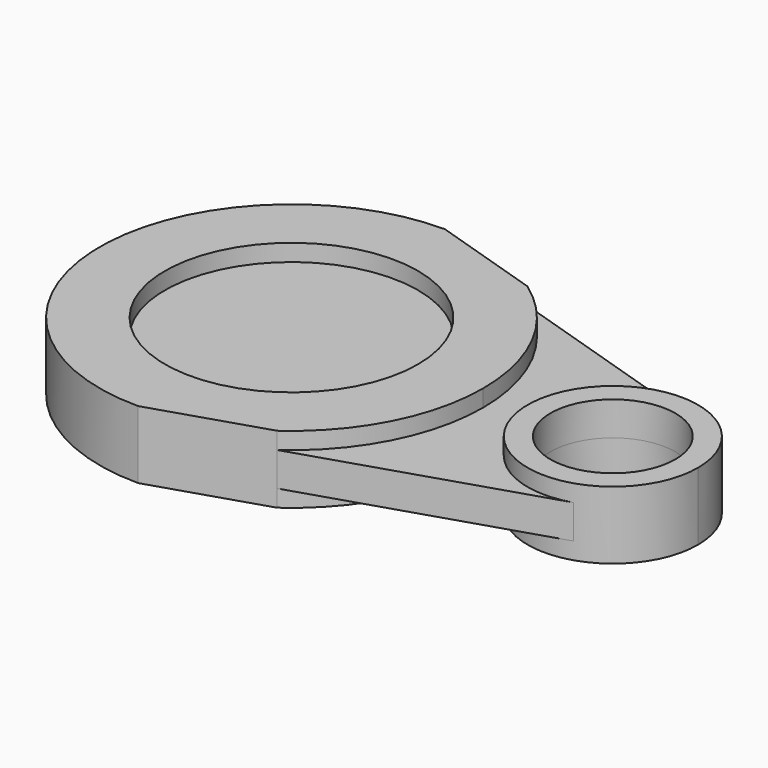
from build123d import *

# Parameters (mm, degrees)
F0_R     = 47.411095877
F1_DEPTH = 12.7
F0_R_2   = 23.4128804589
F2_DEPTH = 6.35


with BuildPart() as f1:
    # F0 (on Top) → F1 (new body, symmetric)
    with BuildSketch(Plane.XY):
        with BuildLine():
            Line((41.5098547303, 58.6180414786), (0, 71.8271733157))
            ThreePointArc((0, 71.8271733157), (-71.8271733157, 0), (0, -71.8271733157))
            Line((0, -71.8271733157), (41.5098547303, -58.6180414786))
            ThreePointArc((41.5098547303, -58.6180414786), (63.7992098562, -32.9970248394), (71.8271733157, 0))
            ThreePointArc((71.8271733157, 0), (63.7992098562, 32.9970248394), (41.5098547303, 58.6180414786))
        make_face()
        Circle(F0_R, mode=Mode.SUBTRACT)
    extrude(amount=F1_DEPTH, both=True)


with BuildPart() as f1b:
    # F0 (on Top) → F1, piece 2 (new body, symmetric)
    with BuildSketch(Plane.XY):
        with BuildLine():
            ThreePointArc((152.353980984, 0), (146.1991452891, 18.845205951), (130.1075988936, 30.4247536263))
            ThreePointArc((130.1075988936, 30.4247536263), (88.4978832347, 0), (130.1075988936, -30.4247536263))
            ThreePointArc((130.1075988936, -30.4247536263), (146.1991452891, -18.845205951), (152.353980984, 0))
        make_face()
        with Locations((120.4259321094, 0)):
            Circle(F0_R_2, mode=Mode.SUBTRACT)
    extrude(amount=F1_DEPTH, both=True)


with BuildPart() as f2:
    # F0 (on Top) → F2 (new body, symmetric)
    with BuildSketch(Plane.XY):
        with BuildLine():
            Line((130.1075988936, 30.4247536263), (41.5098547303, 58.6180414786))
            ThreePointArc((41.5098547303, 58.6180414786), (63.7992098562, 32.9970248394), (71.8271733157, 0))
            ThreePointArc((71.8271733157, 0), (63.7992098562, -32.9970248394), (41.5098547303, -58.6180414786))
            Line((41.5098547303, -58.6180414786), (130.1075988936, -30.4247536263))
            ThreePointArc((130.1075988936, -30.4247536263), (88.4978832347, 0), (130.1075988936, 30.4247536263))
        make_face()
    extrude(amount=F2_DEPTH, both=True)


with BuildPart() as f2b:
    # F0 (on Top) → F2, piece 2 (new body, symmetric)
    with BuildSketch(Plane.XY):
        Circle(F0_R)
    extrude(amount=F2_DEPTH, both=True)


solid = Compound([f1.part, f1b.part, f2.part, f2b.part])
